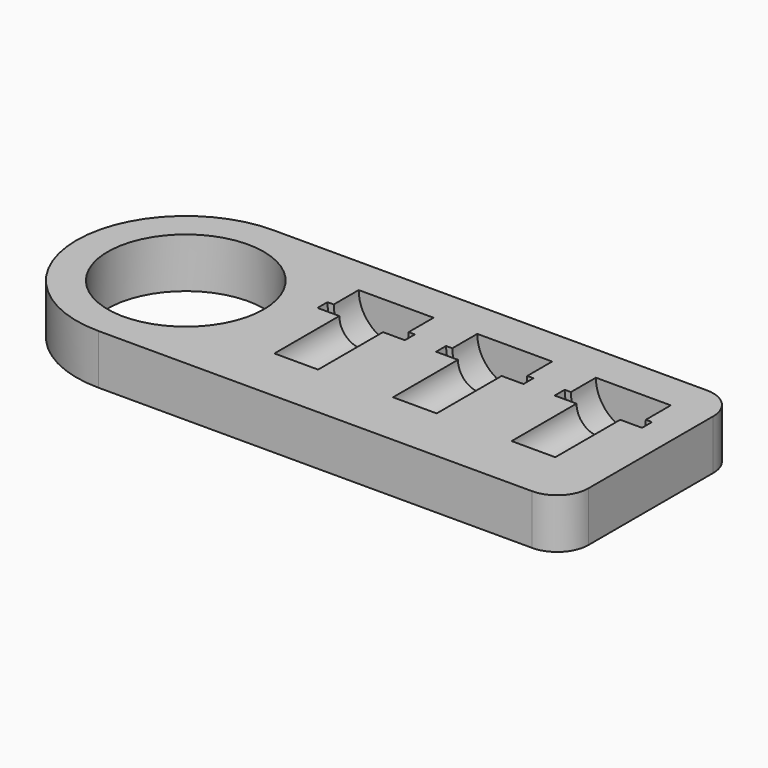
from build123d import *

# Parameters (mm, degrees)
F0_R         = 12.5
F1_DEPTH     = 8
F6_TEXT_SIZE = 5.5555555556
F7_DEPTH     = 1


# Not quite as in the source:
# - Text() gives the source's letters only with a copy of the font that has no kerning and outlines rounded to 1/6400 em; it was checked with that copy


with BuildPart() as f1:
    # F0 (on Top) → F1 (new body)
    with BuildSketch(Plane.XY):
        with BuildLine():
            ThreePointArc((0, 17.5), (5.1256313292, 5.1256313292), (17.5, 0))
            Line((17.5, 0), (87, 0))
            ThreePointArc((87, 0), (90.5355339059, 1.4644660941), (92, 5))
            Line((92, 5), (92, 30))
            ThreePointArc((92, 30), (90.5355339059, 33.5355339059), (87, 35))
            Line((87, 35), (17.5, 35))
            ThreePointArc((17.5, 35), (5.1256313292, 29.8743686708), (0, 17.5))
        make_face()
        with Locations((17.5, 17.5)):
            Circle(F0_R, mode=Mode.SUBTRACT)
    extrude(amount=F1_DEPTH)

    # F2 (on face) → F3 (revolve, cut)
    with BuildSketch(Plane.XY.offset(8)):
        Polygon((42, 22), (42, 9), (45.5, 9), (45.5, 22), (49, 22), (49, 24), (48, 24), (48, 29), (42, 29), (42, 24), align=None)
    revolve(axis=Axis((42, 15.5, 8), (0, 1, 0)), mode=Mode.SUBTRACT)

    # F2 (on face) → F4 (revolve, cut)
    with BuildSketch(Plane.XY.offset(8)):
        Polygon((61, 22), (61, 9), (64.5, 9), (64.5, 22), (68, 22), (68, 24), (67, 24), (67, 29), (61, 29), (61, 24), align=None)
    revolve(axis=Axis((61, 15.5, 8), (0, 1, 0)), mode=Mode.SUBTRACT)

    # F2 (on face) → F5 (revolve, cut)
    with BuildSketch(Plane.XY.offset(8)):
        Polygon((80, 22), (80, 9), (83.5, 9), (83.5, 22), (87, 22), (87, 24), (86, 24), (86, 29), (80, 29), (80, 24), align=None)
    revolve(axis=Axis((80, 15.5, 8), (0, 1, 0)), mode=Mode.SUBTRACT)

    # F6 (on face) → F7 (cut)
    with BuildSketch(Plane(origin=(0, 0, 0), x_dir=(1, 0, 0), z_dir=(0, 0, -1))):
        with Locations((30, -9)):
            Text('798, 883', F6_TEXT_SIZE, font='Open Sans', text_align=(TextAlign.LEFT, TextAlign.BOTTOM))
    extrude(amount=-F7_DEPTH, mode=Mode.SUBTRACT)


solid = f1.part
